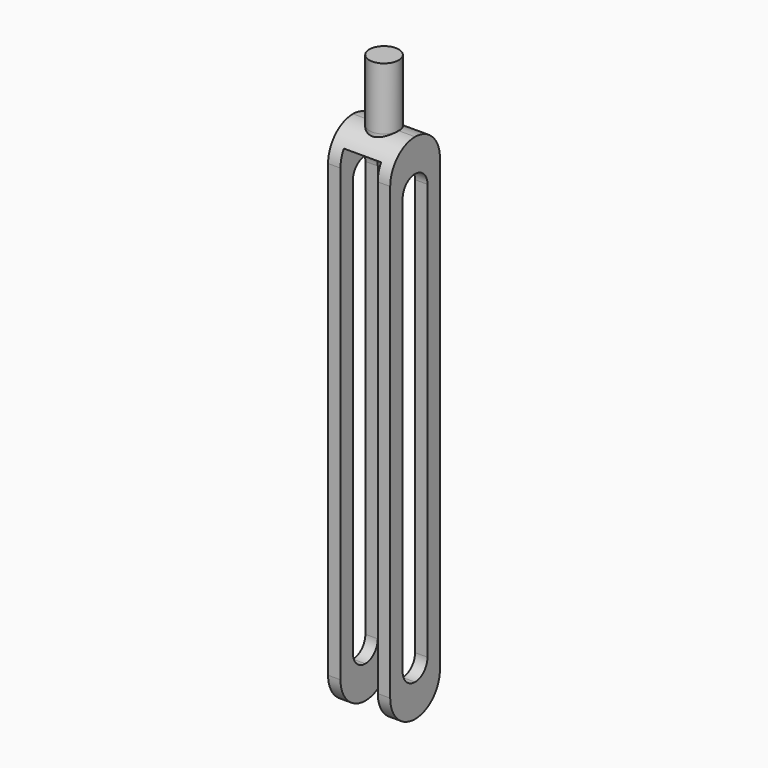
from build123d import *

# Parameters (mm, degrees)
F0_R         = 3
F1_DEPTH     = 12.7
F2_W         = 12.7
F2_H         = 12.7
F3_DEPTH     = 3.175
F4_W         = 2.5373954162
F4_H         = 12.7
F4_W_2       = 2.54
F5_DEPTH     = 101.6
F6_T1_DEPTH  = 34.2873954162
F6_T3_DEPTH  = 34.29
F6_T8_DEPTH  = 44.45
F6_S9_R      = 3
F6_T10_DEPTH = 24
F6_T14_DEPTH = 44.45
F6_S15_R     = 3
F6_T16_DEPTH = 24
F7_W         = 3.175
F7_H         = 91.44
F8_DEPTH     = 25.4
F9_R         = 3.17499


# Not quite as in the source:
# - a fillet or chamfer that OpenCascade refuses, or shapes differently, is made with other operations: its cross-section is extruded or revolved along the edge and cut away or added
# - a fillet or chamfer is up to 0.001 mm smaller than in the source, because OpenCascade refuses the exact size


with BuildPart() as f1:
    # F0 (on Top) → F1 (new body)
    with BuildSketch(Plane.XY):
        Circle(F0_R)
    extrude(amount=F1_DEPTH)

    # F2 (on face) → F3 (join)
    with BuildSketch(Plane(origin=(0, 0, 0), x_dir=(1, 0, 0), z_dir=(0, 0, -1))):
        Rectangle(F2_W, F2_H)
    extrude(amount=F3_DEPTH)

    # F4 (on face) → F5 (join)
    with BuildSketch(Plane(origin=(0, 0, -3.175), x_dir=(1, 0, 0), z_dir=(0, 0, -1))):
        with Locations((-5.0813022919, 0)):
            Rectangle(F4_W, F4_H)
        with Locations((5.08, 0)):
            Rectangle(F4_W_2, F4_H)
    extrude(amount=F5_DEPTH)

    # F6: fillet of radius 6.35 on 6 edges, made by hand

    # F6_s2 → F6_t1 (cut)
    with BuildSketch(Plane.YZ.offset(-22.225)):
        with BuildLine():
            ThreePointArc((-6.35, -98.425), (-4.4901280605, -102.9151280605), (0, -104.775))
            Line((0, -104.775), (-6.35, -104.775))
            Line((-6.35, -104.775), (-6.35, -98.425))
        make_face()
        with BuildLine():
            ThreePointArc((6.35, -98.425), (4.4901280605, -102.9151280605), (0, -104.775))
            Line((0, -104.775), (6.35, -104.775))
            Line((6.35, -104.775), (6.35, -98.425))
        make_face()
    extrude(amount=F6_T1_DEPTH, mode=Mode.SUBTRACT)

    # F6_s4 → F6_t3 (cut)
    with BuildSketch(Plane.YZ.offset(-12.065)):
        with BuildLine():
            ThreePointArc((6.35, -98.425), (4.4901280605, -102.9151280605), (0, -104.775))
            Line((0, -104.775), (6.35, -104.775))
            Line((6.35, -104.775), (6.35, -98.425))
        make_face()
        with BuildLine():
            ThreePointArc((-6.35, -98.425), (-4.4901280605, -102.9151280605), (0, -104.775))
            Line((0, -104.775), (-6.35, -104.775))
            Line((-6.35, -104.775), (-6.35, -98.425))
        make_face()
    extrude(amount=F6_T3_DEPTH, mode=Mode.SUBTRACT)


with BuildPart() as f6_tool6:
    # F6_s7 → F6_t8 (new body)
    with BuildSketch(Plane.YZ.offset(-22.225)):
        with BuildLine():
            ThreePointArc((6.35, -6.35), (4.4901280605, -1.8598719395), (0, 0))
            Line((0, 0), (6.35, 0))
            Line((6.35, 0), (6.35, -6.35))
        make_face()
    extrude(amount=F6_T8_DEPTH)

    # F6_s9 → F6_t10 (cut, symmetric)
    with BuildSketch(Plane.XY.offset(-3.2)):
        Circle(F6_S9_R)
    extrude(amount=F6_T10_DEPTH, both=True, mode=Mode.SUBTRACT)


with BuildPart() as f1_1:
    add(f1.part)

    # F6_t5: cut F6_tool6
    add(f6_tool6.part, mode=Mode.SUBTRACT)


with BuildPart() as f6_tool12:
    # F6_s13 → F6_t14 (new body)
    with BuildSketch(Plane.YZ.offset(22.225)):
        with BuildLine():
            ThreePointArc((0, 0), (-4.4901280605, -1.8598719395), (-6.35, -6.35))
            Line((-6.35, -6.35), (-6.35, 0))
            Line((-6.35, 0), (0, 0))
        make_face()
    extrude(amount=-F6_T14_DEPTH)

    # F6_s15 → F6_t16 (cut, symmetric)
    with BuildSketch(Plane.XY.offset(-3.2)):
        Circle(F6_S15_R)
    extrude(amount=F6_T16_DEPTH, both=True, mode=Mode.SUBTRACT)


with BuildPart() as f1_2:
    add(f1_1.part)

    # F6_t11: cut F6_tool12
    add(f6_tool12.part, mode=Mode.SUBTRACT)

    # F7 (on face) → F8 (cut)
    with BuildSketch(Plane(origin=(-6.35, 0, 0), x_dir=(0, -1, 0), z_dir=(-1, 0, 0))):
        with Locations((1.5875, -52.3875)):
            Rectangle(F7_W, F7_H)
        with Locations((-1.5875, -52.3875)):
            Rectangle(F7_W, F7_H)
    extrude(amount=-F8_DEPTH, mode=Mode.SUBTRACT)

    # F9 (radius 3.175 in the source; OpenCascade refuses exactly that, so slightly less here)
    f9_edges = [f1_2.edges().sort_by_distance(p)[0] for p in [
        (-5.081302, -3.175, -98.1075),
        (-5.081302, -3.175, -6.6675),
        (-5.081302, 3.175, -6.6675),
        (5.08, 3.175, -6.6675),
        (5.08, -3.175, -6.6675),
        (-5.081302, 3.175, -98.1075),
        (5.08, 3.175, -98.1075),
        (5.08, -3.175, -98.1075),
    ]]
    fillet(f9_edges, radius=F9_R)


solid = f1_2.part
